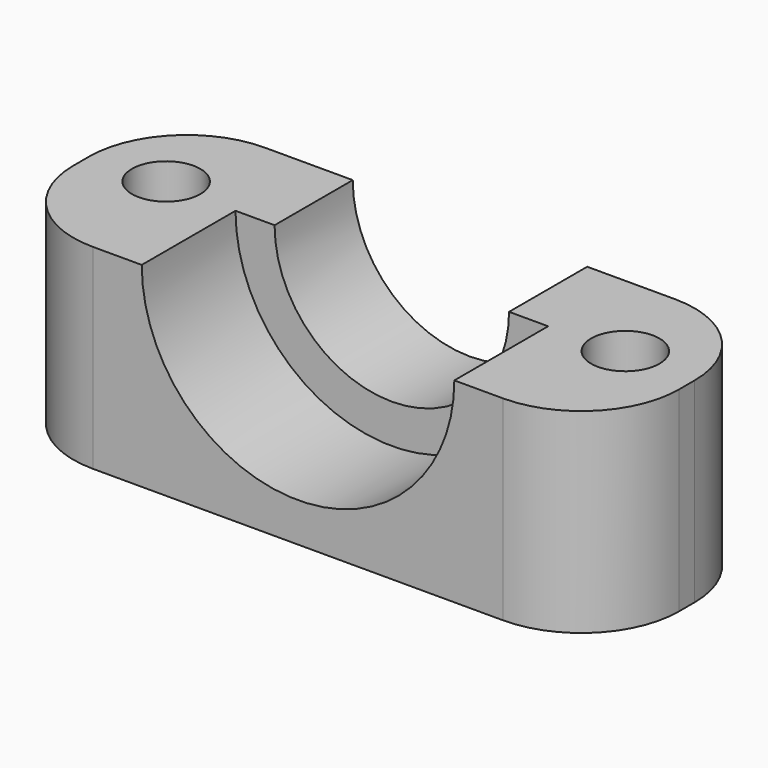
from build123d import *

# Parameters (mm, degrees)
F0_W          = 25
F0_H          = 11
F1_DEPTH      = 10
F2_R          = 8
F3_DEPTH      = 6
F4_R          = 6
F5_DEPTH      = 6
F6_W          = 11
F6_H          = 10
F7_DEPTH      = 3
F8_W          = 11
F8_H          = 10
F9_DEPTH      = 3
F10_R         = 5
F11_R         = 1.75
F12_DEPTH     = 25
F13_TEXT_SIZE = 4.1666666667
F14_DEPTH     = 1


# Not quite as in the source:
# - Text() gives the source's letters only with a copy of the font that has no kerning and outlines rounded to 1/6400 em; it was checked with that copy


with BuildPart() as f1:
    # F0 (on Top) → F1 (new body)
    with BuildSketch(Plane.XY):
        with Locations((12.5, 5.5)):
            Rectangle(F0_W, F0_H)
    extrude(amount=F1_DEPTH)

    # F2 (on face) → F3 (cut)
    with BuildSketch(Plane.XZ):
        with Locations((12.5, 10)):
            Circle(F2_R)
    extrude(amount=-F3_DEPTH, mode=Mode.SUBTRACT)

    # F4 (on face) → F5 (cut)
    with BuildSketch(Plane(origin=(0, 11, 0), x_dir=(-1, 0, 0), z_dir=(0, 1, 0))):
        with Locations((-12.5, 10)):
            Circle(F4_R)
    extrude(amount=-F5_DEPTH, mode=Mode.SUBTRACT)

    # F6 (on face) → F7 (join)
    with BuildSketch(Plane(origin=(0, 0, 0), x_dir=(0, -1, 0), z_dir=(-1, 0, 0))):
        with Locations((-5.5, 5)):
            Rectangle(F6_W, F6_H)
    extrude(amount=F7_DEPTH)

    # F8 (on face) → F9 (join)
    with BuildSketch(Plane.YZ.offset(25)):
        with Locations((5.5, 5)):
            Rectangle(F8_W, F8_H)
    extrude(amount=F9_DEPTH)

    # F10
    f10_edges = [f1.edges().sort_by_distance(p)[0] for p in [
        (28, 11, 5),
        (28, 0, 5),
        (-3, 11, 5),
        (-3, 0, 5),
    ]]
    fillet(f10_edges, radius=F10_R)

    # F11 (on face) → F12 (cut)
    with BuildSketch(Plane.XY.offset(10)):
        with Locations((0.7499999938, 6.25)):
            Circle(F11_R)
        with Locations((24.2499999938, 6.25)):
            Circle(F11_R)
    extrude(amount=-F12_DEPTH, mode=Mode.SUBTRACT)

    # F13 (on face) → F14 (cut)
    with BuildSketch(Plane(origin=(0, 11, 0), x_dir=(-1, 0, 0), z_dir=(0, 1, 0))):
        with Locations((-22.2776692708, 0.25)):
            Text('VOLCANO', F13_TEXT_SIZE, font='Open Sans', text_align=(TextAlign.LEFT, TextAlign.BOTTOM))
    extrude(amount=-F14_DEPTH, mode=Mode.SUBTRACT)


solid = f1.part
